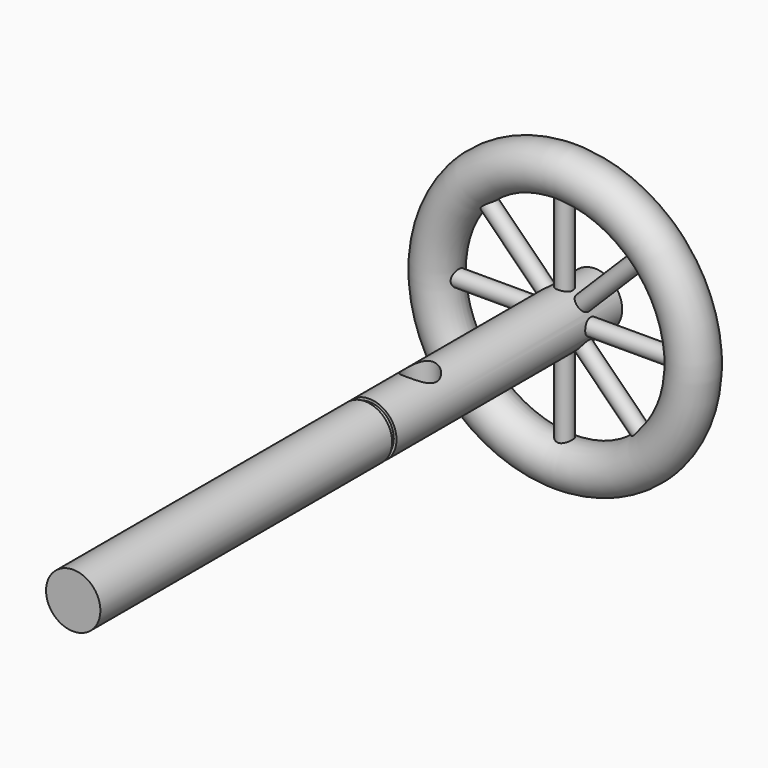
from build123d import *

# Parameters (mm, degrees)
F0_R            = 6.35
F1_DEPTH        = 152.4
F3_R            = 6.35
F3_R_2          = 5.715
F4_DEPTH        = 1.27
F5_R            = 3.8353997866
F6_DEPTH        = 12.7
F7_R            = 1.905
F8_DEPTH        = 25.4
F8_COPIES_COUNT = 8
F11_R           = 5.2430866562


# Not quite as in the source:
# - a pattern or mirror of a feature is missing from the dataset's text; its kind, count and spacing are read off the source's solid


with BuildPart() as f1:
    # F0 (on Front) → F1 (new body)
    with BuildSketch(Plane.XZ):
        Circle(F0_R)
    extrude(amount=F1_DEPTH)

    # F3 (on offset) → F4 (cut)
    with BuildSketch(Plane.XZ.offset(67.183)):
        Circle(F3_R)
        Circle(F3_R_2, mode=Mode.SUBTRACT)
    extrude(amount=-F4_DEPTH, mode=Mode.SUBTRACT)

    # F5 (on Top) → F6 (cut, symmetric)
    with BuildSketch(Plane.XY):
        with Locations((0, -51.0829985142)):
            Circle(F5_R)
    extrude(amount=F6_DEPTH, both=True, mode=Mode.SUBTRACT)

    # F7 (on Top) → F8 (join)
    with BuildSketch(Plane.XY):
        with Locations((0, -8.89)):
            Circle(F7_R)
    f8 = extrude(amount=F8_DEPTH)

    # F8_copies: F8 ×8 about axis
    f8_copies_axis = Axis((0, 0, 0), (0, 1, 0))
    for i in range(1, F8_COPIES_COUNT):
        add(f8.rotate(f8_copies_axis, i * 360 / F8_COPIES_COUNT))

    # F11 (on Top) → F12 (revolve)
    with BuildSketch(Plane.XY):
        with Locations((-29.9154780805, -8.7143657729)):
            Circle(F11_R)
    revolve(axis=Axis((0, -72.4698365666, 0), (0, 1, 0)))


solid = f1.part
